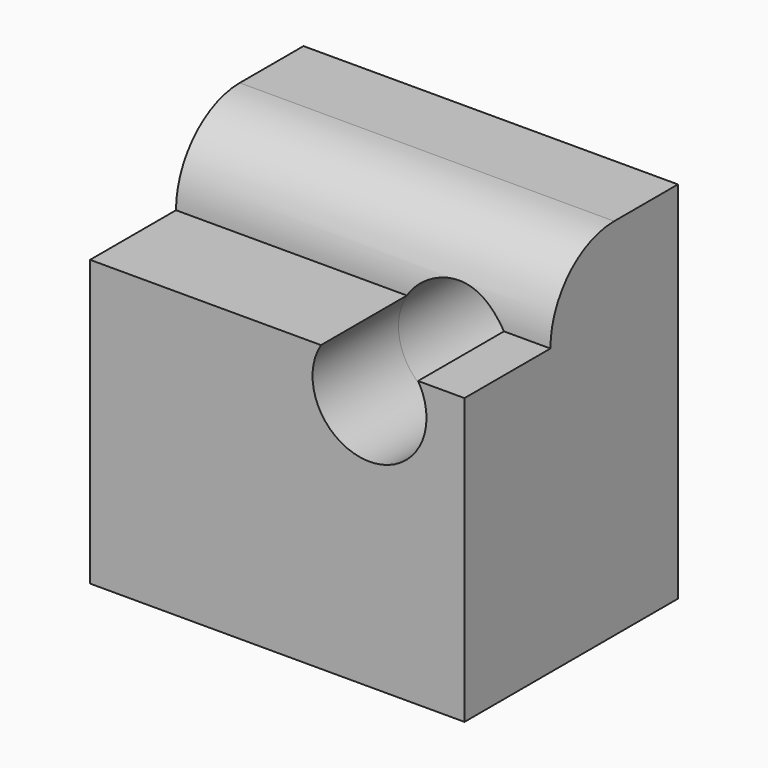
from build123d import *

# Parameters (mm, degrees)
F0_W        = 93.9634628594
F0_H        = 91.5375761688
F1_DEPTH    = 40
F2_R        = 14.2987523314
F3_DEPTH    = 64.5675584674
F4_T1_DEPTH = 193.9634628594
F6_DEPTH    = 26.9540566951


# Not quite as in the source:
# - a fillet or chamfer that OpenCascade refuses, or shapes differently, is made with other operations: its cross-section is extruded or revolved along the edge and cut away or added


with BuildPart() as f1:
    # F0 (on Front) → F1 (new body)
    with BuildSketch(Plane.XZ):
        Rectangle(F0_W, F0_H)
    extrude(amount=F1_DEPTH)

    # F2 (on face) → F3 (cut)
    with BuildSketch(Plane.XZ.offset(40)):
        with Locations((23.1474172324, 18.2785931975)):
            Circle(F2_R)
    extrude(amount=-F3_DEPTH, mode=Mode.SUBTRACT)

    # F4: fillet of radius 20 on 1 edges, made by hand

    # F4_s2 → F4_t1 (cut)
    with BuildSketch(Plane.YZ.offset(-96.9817314297)):
        with BuildLine():
            ThreePointArc((-20, 45.7687880844), (-34.1421356237, 39.9109237081), (-40, 25.7687880844))
            Line((-40, 25.7687880844), (-40, 45.7687880844))
            Line((-40, 45.7687880844), (-20, 45.7687880844))
        make_face()
    extrude(amount=F4_T1_DEPTH, mode=Mode.SUBTRACT)

    # F5 (on face) → F6 (join)
    with BuildSketch(Plane.XZ.offset(40)):
        with BuildLine():
            Line((-46.9817314297, 25.7687880844), (-46.9817314297, -45.7687880844))
            Line((-46.9817314297, -45.7687880844), (46.9817314297, -45.7687880844))
            Line((46.9817314297, -45.7687880844), (46.9817314297, 25.7687880844))
            Line((46.9817314297, 25.7687880844), (35.3273720267, 25.7687880844))
            ThreePointArc((35.3273720267, 25.7687880844), (36.9062775639, 22.1706467187), (37.4461695638, 18.2785931975))
            ThreePointArc((37.4461695638, 18.2785931975), (19.2553637112, 4.5197328659), (10.9674624381, 25.7687880844))
            Line((10.9674624381, 25.7687880844), (-46.9817314297, 25.7687880844))
        make_face()
    extrude(amount=F6_DEPTH)


solid = f1.part
